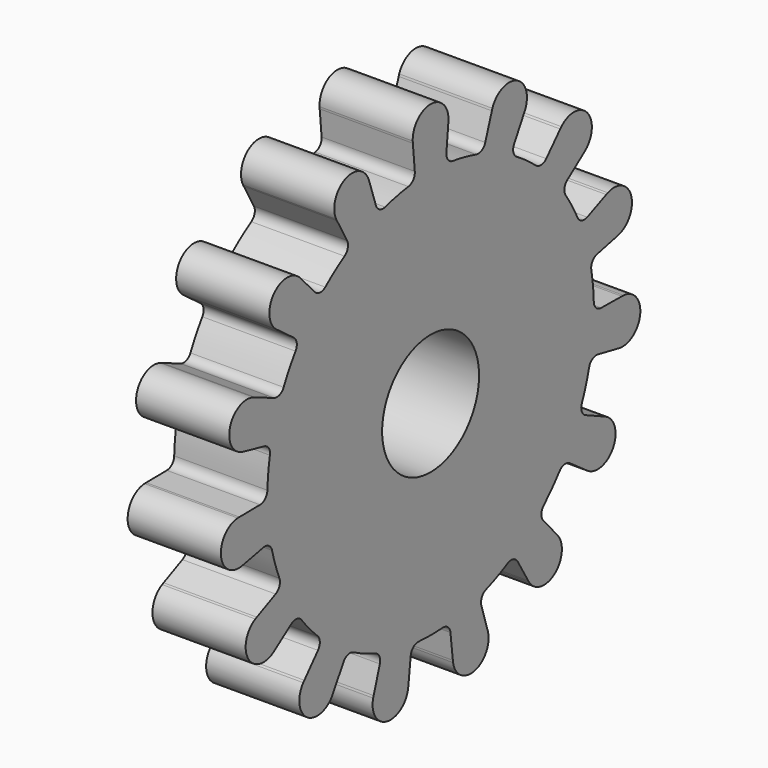
from build123d import *

# Parameters (mm, degrees)
F0_R            = 6.5
F1_DEPTH        = 5
F1_COPIES_COUNT = 15
F2_R            = 1
F3_R            = 1


# Not quite as in the source:
# - a feature of the source that left no trace in its solid (it failed there, or was rolled back) is left out
# - a pattern or mirror of a feature is missing from the dataset's text; its kind, count and spacing are read off the source's solid


with BuildPart() as f1:
    # F0 (on Right) → F1 (new body, symmetric)
    with BuildSketch(Plane.YZ):
        with BuildLine():
            ThreePointArc((-2.0291186985, 21.805794581), (-14.7508016817, -16.1871507607), (21.9, 0))
            ThreePointArc((21.9, 0), (16.1871507607, 14.7508016817), (2.0291186985, 21.805794581))
            ThreePointArc((2.0291186985, 21.805794581), (0, 21.9), (-2.0291186985, 21.805794581))
        make_face()
        Circle(F0_R, mode=Mode.SUBTRACT)
        with BuildLine():
            ThreePointArc((-2.0291186985, 21.805794581), (0, 21.9), (2.0291186985, 21.805794581))
            Line((2.0291186985, 21.805794581), (2.3767920939, 25.5420445339))
            Line((2.3767920939, 25.5420445339), (2.3974176403, 25.7636956522))
            ThreePointArc((2.3974176403, 25.7636956522), (0, 28.275), (-2.3974176403, 25.7636956522))
            Line((-2.3974176403, 25.7636956522), (-2.3767920939, 25.5420445339))
            Line((-2.3767920939, 25.5420445339), (-2.0291186985, 21.805794581))
        make_face()
    extrude(amount=F1_DEPTH, both=True)

    # F1_copies: F1 ×15 about axis
    f1_copies_axis = Axis((0, 0, 0), (1, 0, 0))


with BuildPart() as f1_1:
    add(f1.part)
    for i in range(1, F1_COPIES_COUNT):
        add(f1.part.rotate(f1_copies_axis, i * 360 / F1_COPIES_COUNT))

    # F2
    f2_edges = [f1_1.edges().sort_by_distance(p)[0] for p in [
        (0, -2.029119, 21.805795),
    ]]
    fillet(f2_edges, radius=F2_R)

    # F3
    f3_edges = [f1_1.edges().sort_by_distance(p)[0] for p in [
        (0, 2.029119, 21.805795),
        (0, -7.015524, 20.745902),
        (0, -10.722908, 19.095268),
        (0, -14.847118, 16.098854),
        (0, 7.015524, 20.745902),
        (0, -17.562609, 13.082995),
        (0, 10.722908, 19.095268),
        (0, -20.111511, 8.668168),
        (0, 14.847118, 16.098854),
        (0, -21.365575, 4.808555),
        (0, 17.562609, 13.082995),
        (0, -21.898441, -0.261323),
        (0, 20.111511, 8.668168),
        (0, -21.474239, -4.297329),
        (0, 21.365575, 4.808555),
        (0, -19.898931, -9.145629),
        (0, 21.898441, -0.261323),
        (0, -17.869813, -12.660166),
        (0, 21.474239, -4.297329),
        (0, -14.458716, -16.448572),
        (0, 19.898931, -9.145629),
        (0, -11.175533, -18.833944),
        (0, 17.869813, -12.660166),
        (0, -6.518457, -20.907408),
        (0, 14.458716, -16.448572),
        (0, -2.548902, -21.751163),
        (0, 11.175533, -18.833944),
        (0, 2.548902, -21.751163),
        (0, 6.518457, -20.907408),
    ]]
    fillet(f3_edges, radius=F3_R)

    # F6 (on Front) → F7 (revolve, cut)
    with BuildSketch(Plane.XZ):
        Polygon((-5.1423637196, 8.4322700277), (-2.1835751832, 8.4322700277), (-5.0749732181, 15.1511253789), align=None)
    revolve(axis=Axis((0, 0, 0), (-1, 0, 0)), mode=Mode.SUBTRACT)


solid = f1_1.part
